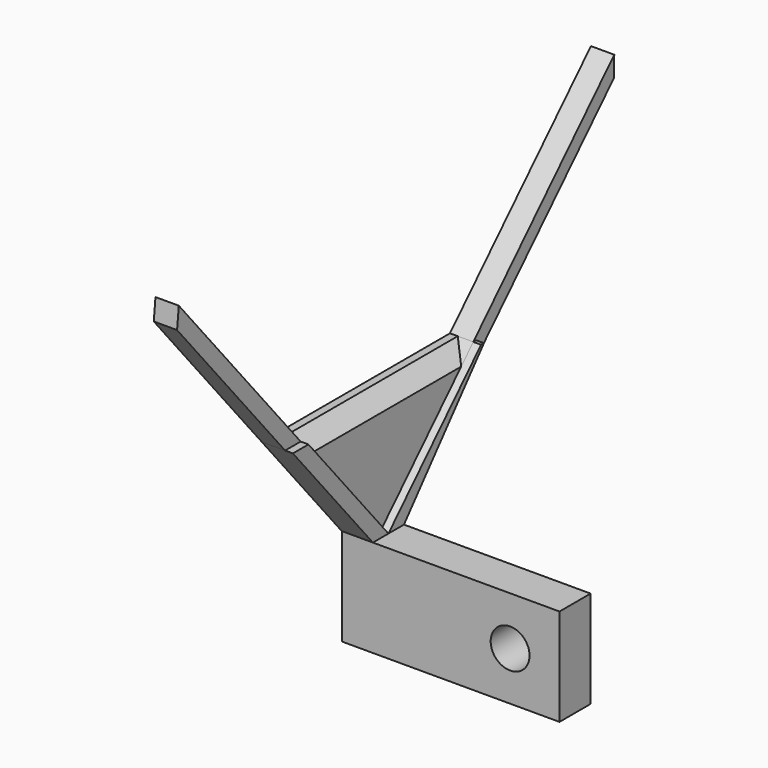
from build123d import *

# Parameters (mm, degrees)
F0_W        = 25
F0_H        = 12.5
F0_R        = 2.5
F1_DEPTH    = 5
F3_DEPTH    = 1
F4_DEPTH    = 3
F5_T4_DEPTH = 38.037750089


# Not quite as in the source:
# - a fillet or chamfer that OpenCascade refuses, or shapes differently, is made with other operations: its cross-section is extruded or revolved along the edge and cut away or added


with BuildPart() as f1:
    # F0 (on Front) → F1 (new body)
    with BuildSketch(Plane.XZ):
        with Locations((-6.15, 0)):
            Rectangle(F0_W, F0_H)
        Circle(F0_R, mode=Mode.SUBTRACT)
    extrude(amount=F1_DEPTH)

    # F2 (on face) → F3 (join)
    with BuildSketch(Plane(origin=(-18.65, 0, 0), x_dir=(0, -1, 0), z_dir=(-1, 0, 0))):
        Polygon((0, 6.25), (0, -6.25), (5, -6.25), (5, 6.25), (2.5, 6.25), align=None)
        Polygon((-12.8557521937, 21.5708888624), (0, 6.25), (2.5, 6.25), (-12.3952659434, 21.5708888624), align=None)
        Polygon((2.5, 6.25), (5, 6.25), (17.8557521937, 21.5708888624), (15.3557521937, 21.5708888624), align=None)
    extrude(amount=-F3_DEPTH)

    # F2 (on face) → F4 (join)
    with BuildSketch(Plane(origin=(-18.65, 0, 0), x_dir=(0, -1, 0), z_dir=(-1, 0, 0))):
        Polygon((0, 6.25), (0, -6.25), (5, -6.25), (5, 6.25), (2.5, 6.25), align=None)
        Polygon((-12.8557521937, 21.5708888624), (0, 6.25), (2.5, 6.25), (-12.3952659434, 21.5708888624), align=None)
        Polygon((-35.0204582804, 42.2711459978), (0, 6.25), (-12.8557521937, 21.5708888624), (-12.3952659434, 21.5708888624), (-35.0532565039, 44.8763173483), align=None)
        Polygon((2.5, 6.25), (5, 6.25), (17.8557521937, 21.5708888624), (15.3557521937, 21.5708888624), align=None)
        Polygon((-12.3952659434, 21.5708888624), (2.5, 6.25), (15.3557521937, 21.5708888624), align=None)
        Polygon((15.3557521937, 21.5708888624), (17.8557521937, 21.5708888624), (35.2253303214, 42.2711459978), (34.9467307814, 44.9185079767), align=None)
    extrude(amount=F4_DEPTH)

    # F5: chamfer of 2 on 1 edges, made by hand


with BuildPart() as f5_tool2:
    # F5_s3 → F5_t4 (new body)
    with BuildSketch(Plane.XZ.offset(20.4991181697)):
        Polygon((-18.65, 19.5708888624), (-20.65, 21.5708888624), (-18.65, 21.5708888624), align=None)
    extrude(amount=-F5_T4_DEPTH)

    split(bisect_by=Plane(origin=(0, -4.4089680227, 4.2864844086), x_dir=(1, 0, 0), z_dir=(0, -0.7169959169, 0.6970773667)), keep=Keep.TOP)

    split(bisect_by=Plane(origin=(0, 1.6104640061, 1.3513397535), x_dir=(1, 0, 0), z_dir=(0, 0.7660444431, 0.6427876097)), keep=Keep.TOP)


with BuildPart() as f1_1:
    add(f1.part)

    # F5_t1: cut F5_tool2
    add(f5_tool2.part, mode=Mode.SUBTRACT)


solid = f1_1.part
